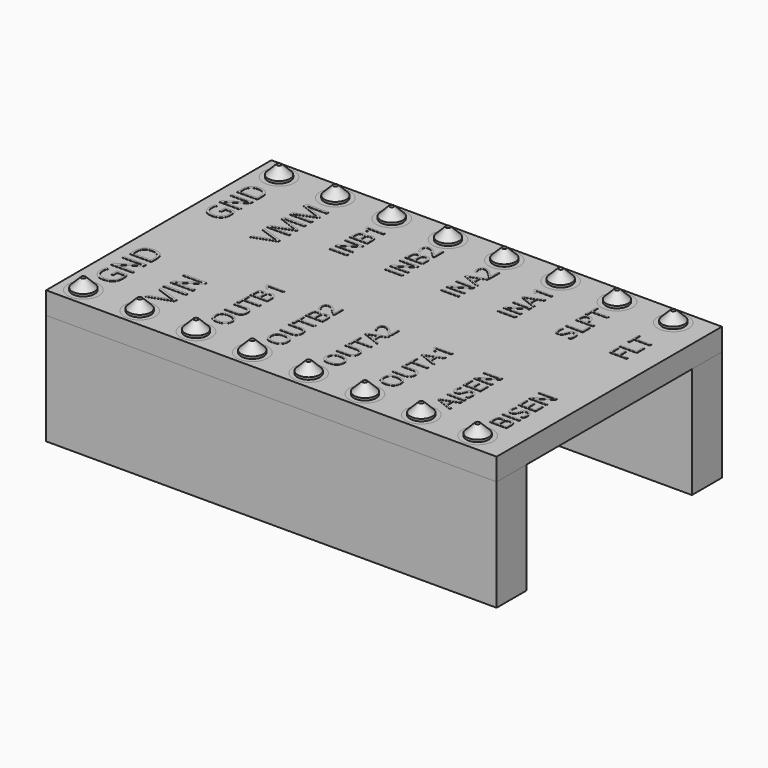
from build123d import *

# Parameters (mm, degrees)
F1_W           = 20.32
F1_H           = 12.7
F1_R           = 0.7
F2_DEPTH       = 1
F1_R_2         = 0.5
F3_DEPTH       = 1
F5_TEXT_SIZE   = 1.3888888889
F5_TEXT_SIZE_2 = 1.303396938
F5_TEXT_SIZE_3 = 1.4307777747
F5_TEXT_SIZE_4 = 1.1111111111
F6_DEPTH       = 0.01
F7_DEPTH       = 1.5
F8_SIZE        = 0.4
F8_2_SIZE      = 0.4
F8_3_SIZE      = 0.4
F8_4_SIZE      = 0.4
F8_5_SIZE      = 0.4
F8_6_SIZE      = 0.4
F8_7_SIZE      = 0.4
F8_8_SIZE      = 0.4
F8_9_SIZE      = 0.4
F8_10_SIZE     = 0.4
F8_11_SIZE     = 0.4
F8_12_SIZE     = 0.4
F8_13_SIZE     = 0.4
F8_14_SIZE     = 0.4
F8_15_SIZE     = 0.4
F8_16_SIZE     = 0.4
F9_W           = 20.32
F9_H           = 1.6922658145
F10_DEPTH      = 5


# Not quite as in the source:
# - Text() gives the source's letters only with a copy of the font that has no kerning and outlines rounded to 1/6400 em; it was checked with that copy


with BuildPart() as f2:
    # F1 (on offset) → F2 (new body)
    with BuildSketch(Plane.XY.offset(5)):
        Rectangle(F1_W, F1_H)
        with Locations((-9.1451881453, -5.5165435188)):
            Circle(F1_R, mode=Mode.SUBTRACT)
        with Locations((-6.6051881453, -5.5165435188)):
            Circle(F1_R, mode=Mode.SUBTRACT)
        with Locations((-4.0651881453, -5.5165435188)):
            Circle(F1_R, mode=Mode.SUBTRACT)
        with Locations((-1.5251881453, -5.5165435188)):
            Circle(F1_R, mode=Mode.SUBTRACT)
        with Locations((1.0148118547, -5.5165435188)):
            Circle(F1_R, mode=Mode.SUBTRACT)
        with Locations((3.5548118547, -5.5165435188)):
            Circle(F1_R, mode=Mode.SUBTRACT)
        with Locations((6.0948118547, -5.5165435188)):
            Circle(F1_R, mode=Mode.SUBTRACT)
        with Locations((8.6348118547, -5.5165435188)):
            Circle(F1_R, mode=Mode.SUBTRACT)
        with Locations((-9.1451881453, 5.5165435188)):
            Circle(F1_R, mode=Mode.SUBTRACT)
        with Locations((-6.6051881453, 5.5165435188)):
            Circle(F1_R, mode=Mode.SUBTRACT)
        with Locations((-4.0651881453, 5.5165435188)):
            Circle(F1_R, mode=Mode.SUBTRACT)
        with Locations((-1.5251881453, 5.5165435188)):
            Circle(F1_R, mode=Mode.SUBTRACT)
        with Locations((1.0148118547, 5.5165435188)):
            Circle(F1_R, mode=Mode.SUBTRACT)
        with Locations((3.5548118547, 5.5165435188)):
            Circle(F1_R, mode=Mode.SUBTRACT)
        with Locations((6.0948118547, 5.5165435188)):
            Circle(F1_R, mode=Mode.SUBTRACT)
        with Locations((8.6348118547, 5.5165435188)):
            Circle(F1_R, mode=Mode.SUBTRACT)
    extrude(amount=F2_DEPTH)


with BuildPart() as f3:
    # F1 (on offset) → F3 (new body)
    with BuildSketch(Plane.XY.offset(5)):
        with Locations((-9.1451881453, 5.5165435188)):
            Circle(F1_R)
        with Locations((-9.1451881453, 5.5165435188)):
            Circle(F1_R_2, mode=Mode.SUBTRACT)
    extrude(amount=F3_DEPTH)


with BuildPart() as f3b:
    # F1 (on offset) → F3, piece 2 (new body)
    with BuildSketch(Plane.XY.offset(5)):
        with Locations((-6.6051881453, 5.5165435188)):
            Circle(F1_R)
        with Locations((-6.6051881453, 5.5165435188)):
            Circle(F1_R_2, mode=Mode.SUBTRACT)
    extrude(amount=F3_DEPTH)


with BuildPart() as f3c:
    # F1 (on offset) → F3, piece 3 (new body)
    with BuildSketch(Plane.XY.offset(5)):
        with Locations((-4.0651881453, 5.5165435188)):
            Circle(F1_R)
        with Locations((-4.0651881453, 5.5165435188)):
            Circle(F1_R_2, mode=Mode.SUBTRACT)
    extrude(amount=F3_DEPTH)


with BuildPart() as f3d:
    # F1 (on offset) → F3, piece 4 (new body)
    with BuildSketch(Plane.XY.offset(5)):
        with Locations((-1.5251881453, 5.5165435188)):
            Circle(F1_R)
        with Locations((-1.5251881453, 5.5165435188)):
            Circle(F1_R_2, mode=Mode.SUBTRACT)
    extrude(amount=F3_DEPTH)


with BuildPart() as f3e:
    # F1 (on offset) → F3, piece 5 (new body)
    with BuildSketch(Plane.XY.offset(5)):
        with Locations((1.0148118547, 5.5165435188)):
            Circle(F1_R)
        with Locations((1.0148118547, 5.5165435188)):
            Circle(F1_R_2, mode=Mode.SUBTRACT)
    extrude(amount=F3_DEPTH)


with BuildPart() as f3f:
    # F1 (on offset) → F3, piece 6 (new body)
    with BuildSketch(Plane.XY.offset(5)):
        with Locations((3.5548118547, 5.5165435188)):
            Circle(F1_R)
        with Locations((3.5548118547, 5.5165435188)):
            Circle(F1_R_2, mode=Mode.SUBTRACT)
    extrude(amount=F3_DEPTH)


with BuildPart() as f3g:
    # F1 (on offset) → F3, piece 7 (new body)
    with BuildSketch(Plane.XY.offset(5)):
        with Locations((6.0948118547, 5.5165435188)):
            Circle(F1_R)
        with Locations((6.0948118547, 5.5165435188)):
            Circle(F1_R_2, mode=Mode.SUBTRACT)
    extrude(amount=F3_DEPTH)


with BuildPart() as f3h:
    # F1 (on offset) → F3, piece 8 (new body)
    with BuildSketch(Plane.XY.offset(5)):
        with Locations((8.6348118547, 5.5165435188)):
            Circle(F1_R)
        with Locations((8.6348118547, 5.5165435188)):
            Circle(F1_R_2, mode=Mode.SUBTRACT)
    extrude(amount=F3_DEPTH)


with BuildPart() as f3i:
    # F1 (on offset) → F3, piece 9 (new body)
    with BuildSketch(Plane.XY.offset(5)):
        with Locations((8.6348118547, -5.5165435188)):
            Circle(F1_R)
        with Locations((8.6348118547, -5.5165435188)):
            Circle(F1_R_2, mode=Mode.SUBTRACT)
    extrude(amount=F3_DEPTH)


with BuildPart() as f3j:
    # F1 (on offset) → F3, piece 10 (new body)
    with BuildSketch(Plane.XY.offset(5)):
        with Locations((6.0948118547, -5.5165435188)):
            Circle(F1_R)
        with Locations((6.0948118547, -5.5165435188)):
            Circle(F1_R_2, mode=Mode.SUBTRACT)
    extrude(amount=F3_DEPTH)


with BuildPart() as f3k:
    # F1 (on offset) → F3, piece 11 (new body)
    with BuildSketch(Plane.XY.offset(5)):
        with Locations((3.5548118547, -5.5165435188)):
            Circle(F1_R)
        with Locations((3.5548118547, -5.5165435188)):
            Circle(F1_R_2, mode=Mode.SUBTRACT)
    extrude(amount=F3_DEPTH)


with BuildPart() as f3l:
    # F1 (on offset) → F3, piece 12 (new body)
    with BuildSketch(Plane.XY.offset(5)):
        with Locations((1.0148118547, -5.5165435188)):
            Circle(F1_R)
        with Locations((1.0148118547, -5.5165435188)):
            Circle(F1_R_2, mode=Mode.SUBTRACT)
    extrude(amount=F3_DEPTH)


with BuildPart() as f3m:
    # F1 (on offset) → F3, piece 13 (new body)
    with BuildSketch(Plane.XY.offset(5)):
        with Locations((-1.5251881453, -5.5165435188)):
            Circle(F1_R)
        with Locations((-1.5251881453, -5.5165435188)):
            Circle(F1_R_2, mode=Mode.SUBTRACT)
    extrude(amount=F3_DEPTH)


with BuildPart() as f3n:
    # F1 (on offset) → F3, piece 14 (new body)
    with BuildSketch(Plane.XY.offset(5)):
        with Locations((-4.0651881453, -5.5165435188)):
            Circle(F1_R)
        with Locations((-4.0651881453, -5.5165435188)):
            Circle(F1_R_2, mode=Mode.SUBTRACT)
    extrude(amount=F3_DEPTH)


with BuildPart() as f3o:
    # F1 (on offset) → F3, piece 15 (new body)
    with BuildSketch(Plane.XY.offset(5)):
        with Locations((-6.6051881453, -5.5165435188)):
            Circle(F1_R)
        with Locations((-6.6051881453, -5.5165435188)):
            Circle(F1_R_2, mode=Mode.SUBTRACT)
    extrude(amount=F3_DEPTH)


with BuildPart() as f3p:
    # F1 (on offset) → F3, piece 16 (new body)
    with BuildSketch(Plane.XY.offset(5)):
        with Locations((-9.1451881453, -5.5165435188)):
            Circle(F1_R)
        with Locations((-9.1451881453, -5.5165435188)):
            Circle(F1_R_2, mode=Mode.SUBTRACT)
    extrude(amount=F3_DEPTH)


with BuildPart() as f6:
    # F5 (on offset) → F6 (new body)
    with BuildSketch(Plane.XY.offset(6)):
        with Locations(Location((-8.6035056713, -4.5572541028), (0, 0, 90))):
            Text('GND', F5_TEXT_SIZE, font='Open Sans', text_align=(TextAlign.LEFT, TextAlign.BOTTOM))
        with Locations(Location((-8.665059876, 1.6299999552), (0, 0, 90))):
            Text('GND', F5_TEXT_SIZE_2, font='Open Sans', text_align=(TextAlign.LEFT, TextAlign.BOTTOM))
        with Locations(Location((-6.0835052282, -4.5572541028), (0, 0, 90))):
            Text('VIN', F5_TEXT_SIZE_3, font='Open Sans', text_align=(TextAlign.LEFT, TextAlign.BOTTOM))
        with Locations(Location((-6.0835052282, 1.2899999274), (0, 0, 90))):
            Text('VMM', F5_TEXT_SIZE, font='Open Sans', text_align=(TextAlign.LEFT, TextAlign.BOTTOM))
        with Locations(Location((-3.5335044757, -4.5572541028), (0, 0, 90))):
            Text('OUTB1', F5_TEXT_SIZE_4, font='Open Sans', text_align=(TextAlign.LEFT, TextAlign.BOTTOM))
        with Locations(Location((-1.0435053062, -4.5572541028), (0, 0, 90))):
            Text('OUTB2', F5_TEXT_SIZE_4, font='Open Sans', text_align=(TextAlign.LEFT, TextAlign.BOTTOM))
        with Locations(Location((4.0499998342, -4.5572541028), (0, 0, 90))):
            Text('OUTA1', F5_TEXT_SIZE_4, font='Open Sans', text_align=(TextAlign.LEFT, TextAlign.BOTTOM))
        with Locations(Location((1.499999975, -4.5572541028), (0, 0, 90))):
            Text('OUTA2', F5_TEXT_SIZE_4, font='Open Sans', text_align=(TextAlign.LEFT, TextAlign.BOTTOM))
        with Locations(Location((6.6099991091, -4.5572541028), (0, 0, 90))):
            Text('AISEN', F5_TEXT_SIZE_4, font='Open Sans', text_align=(TextAlign.LEFT, TextAlign.BOTTOM))
        with Locations(Location((9.0800020844, -4.5572541028), (0, 0, 90))):
            Text('BISEN', F5_TEXT_SIZE_4, font='Open Sans', text_align=(TextAlign.LEFT, TextAlign.BOTTOM))
        with Locations(Location((4.0499998342, 2.2199999075), (0, 0, 90))):
            Text('INA1', F5_TEXT_SIZE_4, font='Open Sans', text_align=(TextAlign.LEFT, TextAlign.BOTTOM))
        with Locations(Location((1.499999975, 2.2199999075), (0, 0, 90))):
            Text('INA2', F5_TEXT_SIZE_4, font='Open Sans', text_align=(TextAlign.LEFT, TextAlign.BOTTOM))
        with Locations(Location((-3.5335044757, 2.2199999075), (0, 0, 90))):
            Text('INB1', F5_TEXT_SIZE_4, font='Open Sans', text_align=(TextAlign.LEFT, TextAlign.BOTTOM))
        with Locations(Location((-1.0435053062, 2.2199999075), (0, 0, 90))):
            Text('INB2', F5_TEXT_SIZE_4, font='Open Sans', text_align=(TextAlign.LEFT, TextAlign.BOTTOM))
        with Locations(Location((6.6099991091, 2.2199999075), (0, 0, 90))):
            Text('SLPT', F5_TEXT_SIZE_4, font='Open Sans', text_align=(TextAlign.LEFT, TextAlign.BOTTOM))
        with Locations(Location((9.0800020844, 2.2199999075), (0, 0, 90))):
            Text('FLT', F5_TEXT_SIZE_4, font='Open Sans', text_align=(TextAlign.LEFT, TextAlign.BOTTOM))
    extrude(amount=F6_DEPTH)


with BuildPart() as f7:
    # F1 (on offset) → F7 (new body)
    with BuildSketch(Plane.XY.offset(5)):
        with Locations((-9.1451881453, 5.5165435188)):
            Circle(F1_R_2)
    extrude(amount=F7_DEPTH)

    # F8#9
    f8_9_edges = [f7.edges().sort_by_distance(p)[0] for p in [
        (-9.645188, 5.516544, 6.5),
    ]]
    chamfer(f8_9_edges, length=F8_9_SIZE)


with BuildPart() as f7b:
    # F1 (on offset) → F7, piece 2 (new body)
    with BuildSketch(Plane.XY.offset(5)):
        with Locations((-6.6051881453, 5.5165435188)):
            Circle(F1_R_2)
    extrude(amount=F7_DEPTH)

    # F8#10
    f8_10_edges = [f7b.edges().sort_by_distance(p)[0] for p in [
        (-7.105188, 5.516544, 6.5),
    ]]
    chamfer(f8_10_edges, length=F8_10_SIZE)


with BuildPart() as f7c:
    # F1 (on offset) → F7, piece 3 (new body)
    with BuildSketch(Plane.XY.offset(5)):
        with Locations((-4.0651881453, 5.5165435188)):
            Circle(F1_R_2)
    extrude(amount=F7_DEPTH)

    # F8#11
    f8_11_edges = [f7c.edges().sort_by_distance(p)[0] for p in [
        (-4.565188, 5.516544, 6.5),
    ]]
    chamfer(f8_11_edges, length=F8_11_SIZE)


with BuildPart() as f7d:
    # F1 (on offset) → F7, piece 4 (new body)
    with BuildSketch(Plane.XY.offset(5)):
        with Locations((-1.5251881453, 5.5165435188)):
            Circle(F1_R_2)
    extrude(amount=F7_DEPTH)

    # F8#12
    f8_12_edges = [f7d.edges().sort_by_distance(p)[0] for p in [
        (-2.025188, 5.516544, 6.5),
    ]]
    chamfer(f8_12_edges, length=F8_12_SIZE)


with BuildPart() as f7e:
    # F1 (on offset) → F7, piece 5 (new body)
    with BuildSketch(Plane.XY.offset(5)):
        with Locations((1.0148118547, 5.5165435188)):
            Circle(F1_R_2)
    extrude(amount=F7_DEPTH)

    # F8#13
    f8_13_edges = [f7e.edges().sort_by_distance(p)[0] for p in [
        (0.514812, 5.516544, 6.5),
    ]]
    chamfer(f8_13_edges, length=F8_13_SIZE)


with BuildPart() as f7f:
    # F1 (on offset) → F7, piece 6 (new body)
    with BuildSketch(Plane.XY.offset(5)):
        with Locations((3.5548118547, 5.5165435188)):
            Circle(F1_R_2)
    extrude(amount=F7_DEPTH)

    # F8#14
    f8_14_edges = [f7f.edges().sort_by_distance(p)[0] for p in [
        (3.054812, 5.516544, 6.5),
    ]]
    chamfer(f8_14_edges, length=F8_14_SIZE)


with BuildPart() as f7g:
    # F1 (on offset) → F7, piece 7 (new body)
    with BuildSketch(Plane.XY.offset(5)):
        with Locations((6.0948118547, 5.5165435188)):
            Circle(F1_R_2)
    extrude(amount=F7_DEPTH)

    # F8#15
    f8_15_edges = [f7g.edges().sort_by_distance(p)[0] for p in [
        (5.594812, 5.516544, 6.5),
    ]]
    chamfer(f8_15_edges, length=F8_15_SIZE)


with BuildPart() as f7h:
    # F1 (on offset) → F7, piece 8 (new body)
    with BuildSketch(Plane.XY.offset(5)):
        with Locations((8.6348118547, 5.5165435188)):
            Circle(F1_R_2)
    extrude(amount=F7_DEPTH)

    # F8#16
    f8_16_edges = [f7h.edges().sort_by_distance(p)[0] for p in [
        (8.134812, 5.516544, 6.5),
    ]]
    chamfer(f8_16_edges, length=F8_16_SIZE)


with BuildPart() as f7i:
    # F1 (on offset) → F7, piece 9 (new body)
    with BuildSketch(Plane.XY.offset(5)):
        with Locations((8.6348118547, -5.5165435188)):
            Circle(F1_R_2)
    extrude(amount=F7_DEPTH)

    # F8#8
    f8_8_edges = [f7i.edges().sort_by_distance(p)[0] for p in [
        (8.134812, -5.516544, 6.5),
    ]]
    chamfer(f8_8_edges, length=F8_8_SIZE)


with BuildPart() as f7j:
    # F1 (on offset) → F7, piece 10 (new body)
    with BuildSketch(Plane.XY.offset(5)):
        with Locations((6.0948118547, -5.5165435188)):
            Circle(F1_R_2)
    extrude(amount=F7_DEPTH)

    # F8#7
    f8_7_edges = [f7j.edges().sort_by_distance(p)[0] for p in [
        (5.594812, -5.516544, 6.5),
    ]]
    chamfer(f8_7_edges, length=F8_7_SIZE)


with BuildPart() as f7k:
    # F1 (on offset) → F7, piece 11 (new body)
    with BuildSketch(Plane.XY.offset(5)):
        with Locations((3.5548118547, -5.5165435188)):
            Circle(F1_R_2)
    extrude(amount=F7_DEPTH)

    # F8#6
    f8_6_edges = [f7k.edges().sort_by_distance(p)[0] for p in [
        (3.054812, -5.516544, 6.5),
    ]]
    chamfer(f8_6_edges, length=F8_6_SIZE)


with BuildPart() as f7l:
    # F1 (on offset) → F7, piece 12 (new body)
    with BuildSketch(Plane.XY.offset(5)):
        with Locations((1.0148118547, -5.5165435188)):
            Circle(F1_R_2)
    extrude(amount=F7_DEPTH)

    # F8#5
    f8_5_edges = [f7l.edges().sort_by_distance(p)[0] for p in [
        (0.514812, -5.516544, 6.5),
    ]]
    chamfer(f8_5_edges, length=F8_5_SIZE)


with BuildPart() as f7m:
    # F1 (on offset) → F7, piece 13 (new body)
    with BuildSketch(Plane.XY.offset(5)):
        with Locations((-1.5251881453, -5.5165435188)):
            Circle(F1_R_2)
    extrude(amount=F7_DEPTH)

    # F8#4
    f8_4_edges = [f7m.edges().sort_by_distance(p)[0] for p in [
        (-2.025188, -5.516544, 6.5),
    ]]
    chamfer(f8_4_edges, length=F8_4_SIZE)


with BuildPart() as f7n:
    # F1 (on offset) → F7, piece 14 (new body)
    with BuildSketch(Plane.XY.offset(5)):
        with Locations((-4.0651881453, -5.5165435188)):
            Circle(F1_R_2)
    extrude(amount=F7_DEPTH)

    # F8#3
    f8_3_edges = [f7n.edges().sort_by_distance(p)[0] for p in [
        (-4.565188, -5.516544, 6.5),
    ]]
    chamfer(f8_3_edges, length=F8_3_SIZE)


with BuildPart() as f7o:
    # F1 (on offset) → F7, piece 15 (new body)
    with BuildSketch(Plane.XY.offset(5)):
        with Locations((-6.6051881453, -5.5165435188)):
            Circle(F1_R_2)
    extrude(amount=F7_DEPTH)

    # F8#2
    f8_2_edges = [f7o.edges().sort_by_distance(p)[0] for p in [
        (-7.105188, -5.516544, 6.5),
    ]]
    chamfer(f8_2_edges, length=F8_2_SIZE)


with BuildPart() as f7p:
    # F1 (on offset) → F7, piece 16 (new body)
    with BuildSketch(Plane.XY.offset(5)):
        with Locations((-9.1451881453, -5.5165435188)):
            Circle(F1_R_2)
    extrude(amount=F7_DEPTH)

    # F8
    f8_edges = [f7p.edges().sort_by_distance(p)[0] for p in [
        (-9.645188, -5.516544, 6.5),
    ]]
    chamfer(f8_edges, length=F8_SIZE)


with BuildPart() as f10:
    # F9 (on Top) → F10 (new body)
    with BuildSketch(Plane.XY):
        with Locations((0, 5.5038670927)):
            Rectangle(F9_W, F9_H)
    extrude(amount=F10_DEPTH)


with BuildPart() as f10b:
    # F9 (on Top) → F10, piece 2 (new body)
    with BuildSketch(Plane.XY):
        with Locations((0, -5.5038670927)):
            Rectangle(F9_W, F9_H)
    extrude(amount=F10_DEPTH)


solid = Compound([f2.part, f3.part, f3b.part, f3c.part, f3d.part, f3e.part, f3f.part, f3g.part, f3h.part, f3i.part, f3j.part, f3k.part, f3l.part, f3m.part, f3n.part, f3o.part, f3p.part, f6.part, f7.part, f7b.part, f7c.part, f7d.part, f7e.part, f7f.part, f7g.part, f7h.part, f7i.part, f7j.part, f7k.part, f7l.part, f7m.part, f7n.part, f7o.part, f7p.part, f10.part, f10b.part])
